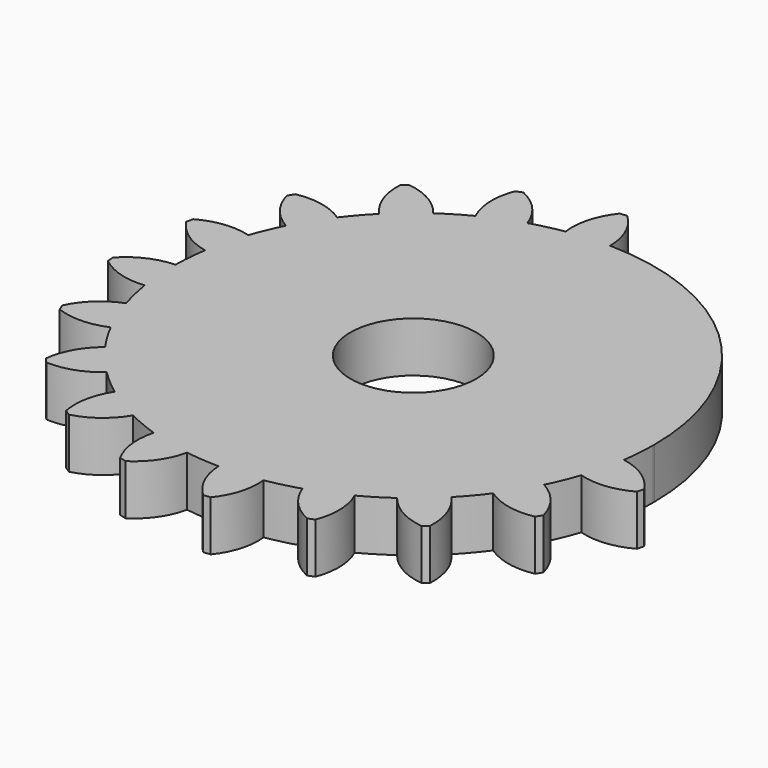
from build123d import *

# Parameters (mm, degrees)
F1_R     = 2.5
F2_DEPTH = 2


with BuildPart() as f2:
    # F1 (on Top) → F2 (new body)
    with BuildSketch(Plane.XY):
        with BuildLine():
            ThreePointArc((-1.5180703499, 9.4623327034), (-0.6836671723, 9.5589160983), (0.1559882342, 9.5820637364))
            ThreePointArc((0.1559882342, 9.5820637364), (-0.0665528354, 10.6175904063), (-0.6817601701, 11.4797736507))
            Line((-0.6817601701, 11.4797736507), (-0.9589212959, 11.4599506957))
            ThreePointArc((-0.9589212959, 11.4599506957), (-1.4451652381, 10.5189901012), (-1.5180703499, 9.4623327034))
        make_face()
        with BuildLine():
            ThreePointArc((9.5830548991, -0.0730518932), (9.5832637245, -0.0365262119), (9.5833333333, 0))
            ThreePointArc((9.5833333333, 0), (6.8313675433, 6.7210635517), (0.1559882342, 9.5820637364))
            ThreePointArc((0.1559882342, 9.5820637364), (-0.6836671723, 9.5589160983), (-1.5180703499, 9.4623327034))
            ThreePointArc((-1.5180703499, 9.4623327034), (-2.1648974057, 9.3356037298), (-2.8014835312, 9.1647131871))
            ThreePointArc((-2.8014835312, 9.1647131871), (-3.5940727612, 8.8838572009), (-4.3589912455, 8.5346044489))
            ThreePointArc((-4.3589912455, 8.5346044489), (-4.9367199241, 8.2139560608), (-5.4909806653, 7.8542605706))
            ThreePointArc((-5.4909806653, 7.8542605706), (-6.1590765347, 7.3420742313), (-6.7796457938, 6.7732326616))
            ThreePointArc((-6.7796457938, 6.7732326616), (-7.2315091117, 6.288525562), (-7.6487959813, 5.7737507579))
            ThreePointArc((-7.6487959813, 5.7737507579), (-8.1264501645, 5.0794768926), (-8.5412652648, 4.3459251552))
            ThreePointArc((-8.5412652648, 4.3459251552), (-8.8219733926, 3.7434026285), (-9.0602402674, 3.1228711268))
            ThreePointArc((-9.0602402674, 3.1228711268), (-9.2997297197, 2.3141531753), (-9.4671849712, 1.4875101679))
            ThreePointArc((-9.4671849712, 1.4875101679), (-9.5476926535, 0.8257377141), (-9.5819980984, 0.159969433))
            ThreePointArc((-9.5819980984, 0.159969433), (-9.5589160983, -0.6836671723), (-9.4617011499, -1.5220016846))
            ThreePointArc((-9.4617011499, -1.5220016846), (-9.3326284876, -2.1776876018), (-9.15817486, -2.8227842658))
            ThreePointArc((-9.15817486, -2.8227842658), (-8.8741934401, -3.6178679586), (-8.5213363969, -4.3848721519))
            ThreePointArc((-8.5213363969, -4.3848721519), (-8.1944813129, -4.9689791497), (-7.8276519112, -5.5288464741))
            ThreePointArc((-7.8276519112, -5.5288464741), (-7.3105655539, -6.1964432588), (-6.7367187038, -6.8159297886))
            ThreePointArc((-6.7367187038, -6.8159297886), (-6.2442438368, -7.2697796861), (-5.7212745776, -7.688126884))
            ThreePointArc((-5.7212745776, -7.688126884), (-5.0222837879, -8.1619203213), (-4.2842988698, -8.5723427937))
            ThreePointArc((-4.2842988698, -8.5723427937), (-3.6754986109, -8.8504795203), (-3.048769233, -9.0854435193))
            ThreePointArc((-3.048769233, -9.0854435193), (-2.2372941238, -9.3185188083), (-1.4084543141, -9.4792686544))
            ThreePointArc((-1.4084543141, -9.4792686544), (-0.7444430671, -9.5543750344), (-0.0768121395, -9.5830254968))
            ThreePointArc((-0.0768121395, -9.5830254968), (0.7666023172, -9.5526226066), (1.6040713479, -9.448133831))
            ThreePointArc((1.6040713479, -9.448133831), (2.2570091235, -9.3137633422), (2.8990260168, -9.1343267914))
            ThreePointArc((2.8990260168, -9.1343267914), (3.6909448761, -8.8440490557), (4.4542736019, -8.4852651377))
            ThreePointArc((4.4542736019, -8.4852651377), (5.0317176792, -8.1561078325), (5.5849573065, -7.7877165885))
            ThreePointArc((5.5849573065, -7.7877165885), (6.2475246624, -7.2669603942), (6.8617811586, -6.6900102473))
            ThreePointArc((6.8617811586, -6.6900102473), (7.3076765099, -6.1998501438), (7.7186345581, -5.6800491491))
            ThreePointArc((7.7186345581, -5.6800491491), (8.1873312003, -4.9807515091), (8.5928495677, -4.2430194537))
            ThreePointArc((8.5928495677, -4.2430194537), (8.864786749, -3.640856173), (9.094586355, -3.0213865706))
            ThreePointArc((9.094586355, -3.0213865706), (9.3244299339, -2.2125289116), (9.4824846776, -1.3866369809))
            ThreePointArc((9.4824846776, -1.3866369809), (9.5553689768, -0.7315746678), (9.5830548991, -0.0730518932))
        make_face()
        Circle(F1_R, mode=Mode.SUBTRACT)
        with BuildLine():
            ThreePointArc((-4.3589912455, 8.5346044489), (-3.5940727612, 8.8838572009), (-2.8014835312, 9.1647131871))
            ThreePointArc((-2.8014835312, 9.1647131871), (-3.3333371832, 10.0728072027), (-4.180233983, 10.6975222247))
            Line((-4.180233983, 10.6975222247), (-4.4377042478, 10.5930219762))
            ThreePointArc((-4.4377042478, 10.5930219762), (-4.6096898874, 9.5557315798), (-4.3589912455, 8.5346044489))
        make_face()
        with BuildLine():
            ThreePointArc((-6.7796457938, 6.7732326616), (-6.1590765347, 7.3420742313), (-5.4909806653, 7.8542605706))
            ThreePointArc((-5.4909806653, 7.8542605706), (-6.2745864185, 8.5442559937), (-7.2657513154, 8.8724690461))
            Line((-7.2657513154, 8.8724690461), (-7.4783277357, 8.6935207164))
            ThreePointArc((-7.4783277357, 8.6935207164), (-7.324432692, 7.6622652015), (-6.7796457938, 6.7732326616))
        make_face()
        with BuildLine():
            ThreePointArc((-8.5412652648, 4.3459251552), (-8.1264501645, 5.0794768926), (-7.6487959813, 5.7737507579))
            ThreePointArc((-7.6487959813, 5.7737507579), (-8.6011727438, 6.1792652434), (-9.6362802326, 6.1832630358))
            Line((-9.6362802326, 6.1832630358), (-9.7831543474, 5.9473833343))
            ThreePointArc((-9.7831543474, 5.9473833343), (-9.3237440683, 5.0213886342), (-8.5412652648, 4.3459251552))
        make_face()
        with BuildLine():
            ThreePointArc((-9.4671849712, 1.4875101679), (-9.2997297197, 2.3141531753), (-9.0602402674, 3.1228711268))
            ThreePointArc((-9.0602402674, 3.1228711268), (-10.0830086743, 3.2081975709), (-11.0597768479, 2.893142415))
            Line((-11.0597768479, 2.893142415), (-11.1265715955, 2.6234208903))
            ThreePointArc((-11.1265715955, 2.6234208903), (-10.4104965865, 1.8894870865), (-9.4671849712, 1.4875101679))
        make_face()
        with BuildLine():
            ThreePointArc((-9.4617011499, -1.5220016846), (-9.5589160983, -0.6836671723), (-9.5819980984, 0.159969433))
            ThreePointArc((-9.5819980984, 0.159969433), (-10.5724717615, -0.0776515645), (-11.3968993944, -0.6758328863))
            Line((-11.3968993944, -0.6758328863), (-11.3770764395, -0.9529940121))
            ThreePointArc((-11.3770764395, -0.9529940121), (-10.4759102131, -1.4277584254), (-9.4617011499, -1.5220016846))
        make_face()
        with BuildLine():
            ThreePointArc((-8.5213363969, -4.3848721519), (-8.8741934401, -3.6178679586), (-9.15817486, -2.8227842658))
            ThreePointArc((-9.15817486, -2.8227842658), (-10.0198511487, -3.3547436632), (-10.6146479684, -4.1743066993))
            Line((-10.6146479684, -4.1743066993), (-10.5101477199, -4.431776964))
            ThreePointArc((-10.5101477199, -4.431776964), (-9.5111048977, -4.6049448476), (-8.5213363969, -4.3848721519))
        make_face()
        with BuildLine():
            ThreePointArc((-6.7367187038, -6.8159297886), (-7.3105655539, -6.1964432588), (-7.8276519112, -5.5288464741))
            ThreePointArc((-7.8276519112, -5.5288464741), (-8.4789113447, -6.2997024123), (-8.7895947898, -7.2598240316))
            Line((-8.7895947898, -7.2598240316), (-8.6106464602, -7.472400452))
            ThreePointArc((-8.6106464602, -7.472400452), (-7.6089149783, -7.3290474265), (-6.7367187038, -6.8159297886))
        make_face()
        with BuildLine():
            ThreePointArc((-5.8645090781, -9.7772270637), (-4.9554278588, -9.3308225469), (-4.2842988698, -8.5723427937))
            ThreePointArc((-4.2842988698, -8.5723427937), (-5.0222837879, -8.1619203213), (-5.7212745776, -7.688126884))
            ThreePointArc((-5.7212745776, -7.688126884), (-6.1017529133, -8.6219729099), (-6.1003887796, -9.6303529489))
            Line((-6.1003887796, -9.6303529489), (-5.8645090781, -9.7772270637))
        make_face()
        with BuildLine():
            ThreePointArc((-2.5405466341, -11.1206443117), (-1.8118261707, -10.4121564714), (-1.4084543141, -9.4792686544))
            ThreePointArc((-1.4084543141, -9.4792686544), (-2.2372941238, -9.3185188083), (-3.048769233, -9.0854435193))
            ThreePointArc((-3.048769233, -9.0854435193), (-3.1234277994, -10.0931414551), (-2.8102681588, -11.0538495641))
            Line((-2.8102681588, -11.0538495641), (-2.5405466341, -11.1206443117))
        make_face()
        with BuildLine():
            ThreePointArc((1.0358682683, -11.3711491557), (1.511723831, -10.4663000259), (1.6040713479, -9.448133831))
            ThreePointArc((1.6040713479, -9.448133831), (0.7666023172, -9.5526226066), (-0.0768121395, -9.5830254968))
            ThreePointArc((-0.0768121395, -9.5830254968), (0.1619836909, -10.5697046278), (0.7587071426, -11.3909721106))
            Line((0.7587071426, -11.3909721106), (1.0358682683, -11.3711491557))
        make_face()
        with BuildLine():
            ThreePointArc((4.5146512203, -10.5042204361), (4.6873777355, -9.4886745278), (4.4542736019, -8.4852651377))
            ThreePointArc((4.4542736019, -8.4852651377), (3.6909448761, -8.8440490557), (2.8990260168, -9.1343267914))
            ThreePointArc((2.8990260168, -9.1343267914), (3.4311318006, -10.0069084012), (4.2571809555, -10.6087206847))
            Line((4.2571809555, -10.6087206847), (4.5146512203, -10.5042204361))
        make_face()
        with BuildLine():
            ThreePointArc((7.5552747082, -8.6047191764), (7.402679542, -7.5770444213), (6.8617811586, -6.6900102473))
            ThreePointArc((6.8617811586, -6.6900102473), (6.2475246624, -7.2669603942), (5.5849573065, -7.7877165885))
            ThreePointArc((5.5849573065, -7.7877165885), (6.3637064246, -8.4623949716), (7.3426982879, -8.783667506))
            Line((7.3426982879, -8.783667506), (7.5552747082, -8.6047191764))
        make_face()
        with BuildLine():
            ThreePointArc((9.8601013199, -5.8585817943), (9.3917672324, -4.921145269), (8.5928495677, -4.2430194537))
            ThreePointArc((8.5928495677, -4.2430194537), (8.1873312003, -4.9807515091), (7.7186345581, -5.6800491491))
            ThreePointArc((7.7186345581, -5.6800491491), (8.673892426, -6.0895890492), (9.7132272051, -6.0944614958))
            Line((9.7132272051, -6.0944614958), (9.8601013199, -5.8585817943))
        make_face()
        with BuildLine():
            ThreePointArc((11.2035185679, -2.5346193503), (10.4614187824, -1.7830993547), (9.4824846776, -1.3866369809))
            ThreePointArc((9.4824846776, -1.3866369809), (9.3244299339, -2.2125289116), (9.094586355, -3.0213865706))
            ThreePointArc((9.094586355, -3.0213865706), (10.1378657141, -3.1218388518), (11.1367238204, -2.804340875))
            Line((11.1367238204, -2.804340875), (11.2035185679, -2.5346193503))
        make_face()
    extrude(amount=F2_DEPTH)


solid = f2.part
